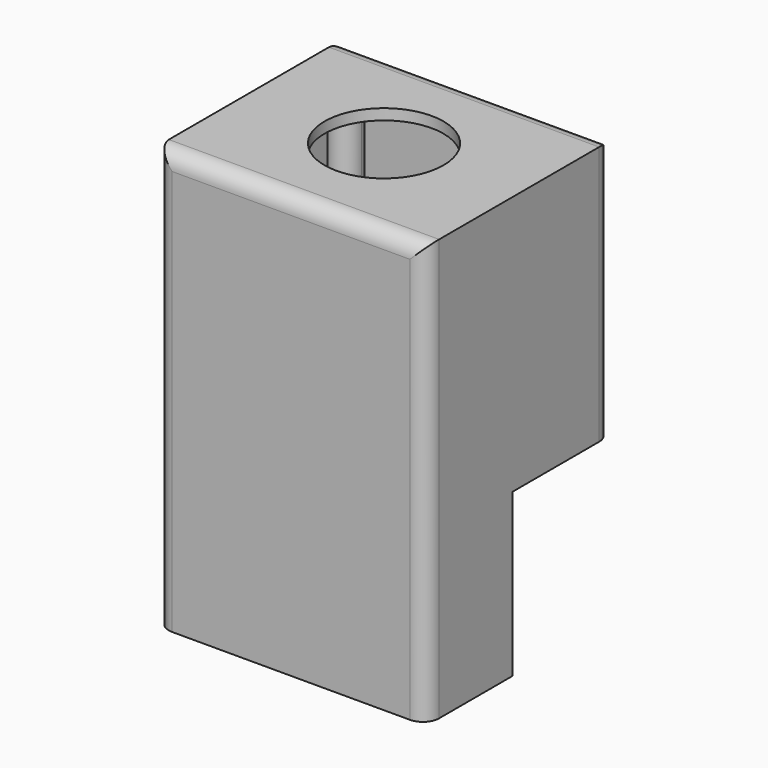
from build123d import *

# Parameters (mm, degrees)
F0_W      = 50
F0_H      = 43
F0_R      = 1.5
F1_DEPTH  = 78
F3_T      = -2
F2_R      = 11
F4_DEPTH  = 3.1
F5_R      = 3
F6_R      = 1.5
F7_DEPTH  = 75
F8_DEPTH  = 40
F9_W      = 50
F9_H      = 23
F10_DEPTH = 30


# Not quite as in the source:
# - a feature names something its author has since deleted; it is built from what else it names


with BuildPart() as f1:
    # F0 (on Top) → F1 (new body)
    with BuildSketch(Plane.XY):
        with Locations((-9.0278687937, 4.7237686813)):
            Rectangle(F0_W, F0_H)
        with Locations((-31.0278687937, -13.7762313187)):
            Circle(F0_R, mode=Mode.SUBTRACT)
        with Locations((12.9721312063, -13.7762313187)):
            Circle(F0_R, mode=Mode.SUBTRACT)
        with Locations((-31.0278687937, 23.2237686813)):
            Circle(F0_R, mode=Mode.SUBTRACT)
        with Locations((12.9721312063, 23.2237686813)):
            Circle(F0_R, mode=Mode.SUBTRACT)
        with Locations((12.9721312063, 23.2237686813)):
            Circle(F0_R)
        with Locations((12.9721312063, -13.7762313187)):
            Circle(F0_R)
        with Locations((-31.0278687937, -13.7762313187)):
            Circle(F0_R)
        with Locations((-31.0278687937, 23.2237686813)):
            Circle(F0_R)
    extrude(amount=F1_DEPTH)

    # F3
    f3_openings = [f1.faces().sort_by_distance(p)[0] for p in [
        (-9.027869, 4.723769, 0),
    ]]
    offset(amount=F3_T, openings=f3_openings)

    # F2 (on face) → F4 (cut)
    with BuildSketch(Plane.XY.offset(78)):
        with Locations((-9.0278687937, 4.7237686813)):
            Circle(F2_R)
    extrude(amount=-F4_DEPTH, mode=Mode.SUBTRACT)

    # F5
    f5_edges = [f1.edges().sort_by_distance(p)[0] for p in [
        (15.972131, 26.223769, 39),
        (-9.027869, 26.223769, 78),
        (-34.027869, 26.223769, 39),
        (15.972131, -16.776231, 39),
        (-9.027869, -16.776231, 78),
        (-34.027869, -16.776231, 39),
    ]]
    fillet(f5_edges, radius=F5_R)

    # F6 (on face) → F7 (join)
    with BuildSketch(Plane.XY):
        with BuildLine():
            ThreePointArc((12.9721312104, -16.7762313187), (15.0934515513, -15.8975516608), (15.9721312063, -13.7762313187))
            ThreePointArc((15.9721312063, -13.7762313187), (10.8508108613, -11.6549109766), (12.9721312104, -16.7762313187))
        make_face()
        with Locations((12.9721312063, -13.7762313187)):
            Circle(F6_R, mode=Mode.SUBTRACT)
        with BuildLine():
            ThreePointArc((12.9721312063, 26.2237686813), (10.8508108627, 21.1024483377), (15.9721312063, 23.2237686813))
            ThreePointArc((15.9721312063, 23.2237686813), (15.0934515498, 25.3450890248), (12.9721312063, 26.2237686813))
        make_face()
        with Locations((12.9721312063, 23.2237686813)):
            Circle(F6_R, mode=Mode.SUBTRACT)
        with BuildLine():
            ThreePointArc((-34.0278687937, -13.776231286), (-33.1491891488, -15.8975516507), (-31.0278687937, -16.7762313187))
            ThreePointArc((-31.0278687937, -16.7762313187), (-28.9065484502, -15.8975516623), (-28.0278687937, -13.7762313187))
            ThreePointArc((-28.0278687937, -13.7762313187), (-31.0278687774, -10.7762313187), (-34.0278687937, -13.776231286))
        make_face()
        with Locations((-31.0278687937, -13.7762313187)):
            Circle(F6_R, mode=Mode.SUBTRACT)
        with BuildLine():
            ThreePointArc((-28.0278687937, 23.2237686813), (-28.9065484366, 25.3450890113), (-31.0278687555, 26.2237686813))
            ThreePointArc((-31.0278687555, 26.2237686813), (-33.1491891237, 25.3450890384), (-34.0278687937, 23.2237686813))
            ThreePointArc((-34.0278687937, 23.2237686813), (-31.0278687937, 20.2237686813), (-28.0278687937, 23.2237686813))
        make_face()
        with Locations((-31.0278687937, 23.2237686813)):
            Circle(F6_R, mode=Mode.SUBTRACT)
    extrude(amount=F7_DEPTH)

    # F0 (on Top) → F8 (cut)
    with BuildSketch(Plane.XY):
        with Locations((-31.0278687937, 23.2237686813)):
            Circle(F0_R)
        with Locations((12.9721312063, 23.2237686813)):
            Circle(F0_R)
        with Locations((-31.0278687937, -13.7762313187)):
            Circle(F0_R)
        with Locations((12.9721312063, -13.7762313187)):
            Circle(F0_R)
    extrude(amount=F8_DEPTH, mode=Mode.SUBTRACT)

    # F9 (on Top) → F10 (cut)
    with BuildSketch(Plane.XY):
        with Locations((-9.0278687937, 14.7237686813)):
            Rectangle(F9_W, F9_H)
    extrude(amount=F10_DEPTH, mode=Mode.SUBTRACT)


solid = f1.part
